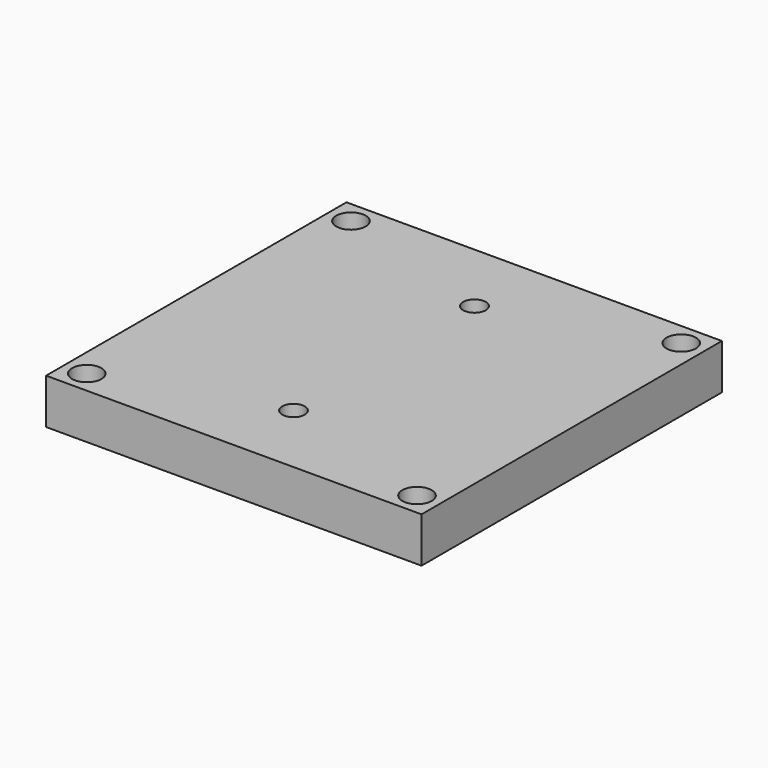
from build123d import *

# Parameters (mm, degrees)
F0_W           = 83
F0_H           = 83
F1_DEPTH       = 10
F2_R           = 3.25
F3_DEPTH       = 10
F5_D           = 5
F5_DEPTH       = 15
F5_CBORE_D     = 11.25
F5_CBORE_DEPTH = 6
F5_TIP         = 1.5021515476


with BuildPart() as f1:
    # F0 (on Top) → F1 (new body)
    with BuildSketch(Plane.XY):
        Rectangle(F0_W, F0_H)
    extrude(amount=F1_DEPTH)

    # F2 (on face) → F3 (cut, through all)
    with BuildSketch(Plane.XY.offset(10)):
        with Locations((-36.5, 36.5)):
            Circle(F2_R)
        with Locations((-36.5, -36.5)):
            Circle(F2_R)
        with Locations((36.5, -36.5)):
            Circle(F2_R)
        with Locations((36.5, 36.5)):
            Circle(F2_R)
    extrude(amount=-F3_DEPTH, mode=Mode.SUBTRACT)

    # F5
    with Locations(Plane(origin=(0, 0, 0), x_dir=(1, 0, 0), z_dir=(0, 0, -1))):
        with Locations((0, -25), (0, 25)):
            CounterBoreHole(F5_D / 2, F5_CBORE_D / 2, F5_CBORE_DEPTH, depth=F5_DEPTH)
            with Locations((0, 0, -(F5_DEPTH + F5_TIP / 2))):  # 118° drill point
                Cone(0, F5_D / 2, F5_TIP, mode=Mode.SUBTRACT)


solid = f1.part
